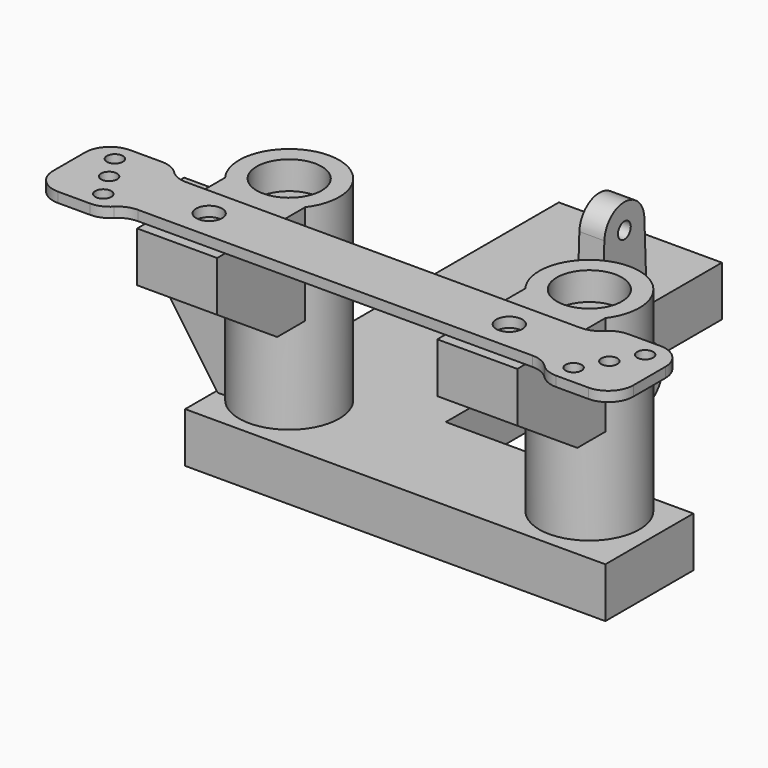
from build123d import *

# Parameters (mm, degrees)
F0_W         = 84
F0_H         = 22
F0_R         = 3
F1_DEPTH     = 10
F3_DEPTH     = 3.2
F6_R         = 4.15
F7_DEPTH     = 20
F8_T1_DEPTH  = 93.5140157162
F9_R         = 7.1
F10_DEPTH    = 12
F12_R        = 1.6
F12_R_2      = 2.6
F13_DEPTH    = 2
F14_T1_DEPTH = 27
F14_T3_DEPTH = 24.9128784748
F15_R        = 5
F17_DEPTH    = 5
F18_R        = 1.6
F19_DEPTH    = 5
F20_R        = 6
F20_R_2      = 1.6
F21_DEPTH    = 3
F22_R        = 4
F23_DEPTH    = 4
F25_DEPTH    = 20
F26_D        = 3.2
F28_W        = 32.6
F28_H        = 69
F29_DEPTH    = 10


# Not quite as in the source:
# - a fillet or chamfer that OpenCascade refuses, or shapes differently, is made with other operations: its cross-section is extruded or revolved along the edge and cut away or added


with BuildPart() as f1:
    # F0 (on Top) → F1 (new body)
    with BuildSketch(Plane.XY):
        Rectangle(F0_W, F0_H)
        with Locations((-30, 0)):
            Circle(F0_R, mode=Mode.SUBTRACT)
        with Locations((30, 0)):
            Circle(F0_R, mode=Mode.SUBTRACT)
    extrude(amount=F1_DEPTH)

    # F2 (on face) → F3 (cut)
    with BuildSketch(Plane.XY.offset(10)):
        Polygon((-25, -2.8867513459), (-25, 2.8867513459), (-30, 5.7735026919), (-35, 2.8867513459), (-35, -2.8867513459), (-30, -5.7735026919), align=None)
        Polygon((25, 2.8867513459), (25, -2.8867513459), (30, -5.7735026919), (35, -2.8867513459), (35, 2.8867513459), (30, 5.7735026919), align=None)
    extrude(amount=-F3_DEPTH, mode=Mode.SUBTRACT)

    # F28 (on face) → F29 (join)
    with BuildSketch(Plane.XY):
        with Locations((-23.8, 45.5)):
            Rectangle(F28_W, F28_H)
    extrude(amount=F29_DEPTH)


with BuildPart() as f5:
    # F4 (on Front) → F5 (revolve)
    with BuildSketch(Plane.XZ):
        Polygon((-40, 50), (-40, 11), (-36.5, 11), (-36.5, 16.6), (-33, 16.6), (-33, 44.4), (-36.5, 44.4), (-36.5, 50), align=None)
    revolve(axis=Axis((-30, 0, 5.9249366093), (0, 0, -1)))

    # F6 (on face) → F7 (join)
    with BuildSketch(Plane.XY.offset(50)):
        with BuildLine():
            ThreePointArc((-22, -6), (-30, -10), (-38, -6))
            Line((-38, -6), (-38, -28))
            Line((-38, -28), (-22, -28))
            Line((-22, -28), (-22, -6))
        make_face()
        with Locations((-30, -20)):
            Circle(F6_R, mode=Mode.SUBTRACT)
    extrude(amount=-F7_DEPTH)

    # F8: chamfer of 10 x 15 on 1 edges, made by hand

    # F8_s2 → F8_t1 (cut)
    with BuildSketch(Plane.YZ.offset(-76.7570078581)):
        Polygon((-13, 30), (-28, 40), (-28, 30), align=None)
    extrude(amount=F8_T1_DEPTH, mode=Mode.SUBTRACT)

    # F9 (on face) → F10 (cut)
    with BuildSketch(Plane(origin=(0, 0, 30), x_dir=(1, 0, 0), z_dir=(0, 0, -1))):
        with Locations((-30, 20)):
            Circle(F9_R)
    extrude(amount=-F10_DEPTH, mode=Mode.SUBTRACT)


with BuildPart() as f11_1:
    # F11: copy of F5
    add(f5.part.moved(Location((60, 0, 0))))


with BuildPart() as f13:
    # F12 (on face) → F13 (new body)
    with BuildSketch(Plane.XY.offset(50)):
        Polygon((0, -26), (42, -26), (42, -29), (58, -29), (58, -11), (42, -11), (42, -14), (0, -14), (-42, -14), (-42, -11), (-58, -11), (-58, -29), (-42, -29), (-42, -26), align=None)
        with Locations((-47, -25.1961524227)):
            Circle(F12_R, mode=Mode.SUBTRACT)
        with Locations((47, -25.1961524227)):
            Circle(F12_R, mode=Mode.SUBTRACT)
        with Locations((-50, -20)):
            Circle(F12_R, mode=Mode.SUBTRACT)
        with Locations((-30, -20)):
            Circle(F12_R_2, mode=Mode.SUBTRACT)
        with Locations((-53, -14.8038475773)):
            Circle(F12_R, mode=Mode.SUBTRACT)
        with Locations((30, -20)):
            Circle(F12_R_2, mode=Mode.SUBTRACT)
        with Locations((50, -20)):
            Circle(F12_R, mode=Mode.SUBTRACT)
        with Locations((53, -14.8038475773)):
            Circle(F12_R, mode=Mode.SUBTRACT)
    extrude(amount=F13_DEPTH)

    # F14: fillet of radius 5 on 8 edges, made by hand

    # F14_s2 → F14_t1 (cut)
    with BuildSketch(Plane.XY.offset(37.5)):
        with BuildLine():
            ThreePointArc((-53, -29), (-56.5355339059, -27.5355339059), (-58, -24))
            Line((-58, -24), (-58, -29))
            Line((-58, -29), (-53, -29))
        make_face()
        with BuildLine():
            ThreePointArc((-58, -16), (-56.5355339059, -12.4644660941), (-53, -11))
            Line((-53, -11), (-58, -11))
            Line((-58, -11), (-58, -16))
        make_face()
        with BuildLine():
            ThreePointArc((58, -24), (56.5355339059, -27.5355339059), (53, -29))
            Line((53, -29), (58, -29))
            Line((58, -29), (58, -24))
        make_face()
        with BuildLine():
            ThreePointArc((53, -11), (56.5355339059, -12.4644660941), (58, -16))
            Line((58, -16), (58, -11))
            Line((58, -11), (53, -11))
        make_face()
    extrude(amount=F14_T1_DEPTH, mode=Mode.SUBTRACT)

    # F14_s4 → F14_t3 (cut)
    with BuildSketch(Plane.XY.offset(38.5435607626)):
        with BuildLine():
            ThreePointArc((-46.582575695, -29), (-43.8439629074, -28.1833001327), (-42, -26))
            Line((-42, -26), (-42, -29))
            Line((-42, -29), (-46.582575695, -29))
        make_face()
        with BuildLine():
            ThreePointArc((-46.582575695, -11), (-43.8439629074, -11.8166998673), (-42, -14))
            Line((-42, -14), (-42, -11))
            Line((-42, -11), (-46.582575695, -11))
        make_face()
        with BuildLine():
            ThreePointArc((46.582575695, -29), (43.8439629074, -28.1833001327), (42, -26))
            Line((42, -26), (42, -29))
            Line((42, -29), (46.582575695, -29))
        make_face()
        with BuildLine():
            ThreePointArc((42, -14), (43.8439629074, -11.8166998673), (46.582575695, -11))
            Line((46.582575695, -11), (42, -11))
            Line((42, -11), (42, -14))
        make_face()
    extrude(amount=F14_T3_DEPTH, mode=Mode.SUBTRACT)

    # F15
    f15_edges = [f13.edges().sort_by_distance(p)[0] for p in [
        (42, -26, 51),
        (42, -14, 51),
        (-42, -14, 51),
        (-42, -26, 51),
    ]]
    fillet(f15_edges, radius=F15_R)


with BuildPart() as f5_1:
    add(f5.part)

    # F16 (on Front) → F17 (join, symmetric)
    with BuildSketch(Plane.XZ):
        Polygon((-40, 32.8592599663), (-45, 40), (-55, 40), (-55, 32), (-40.2956416976, 11), (-37, 11), (-37, 32.8592599663), align=None)
    extrude(amount=F17_DEPTH, both=True)

    # F24 (on face) → F25 (cut)
    with BuildSketch(Plane(origin=(0, 0, 11), x_dir=(1, 0, 0), z_dir=(0, 0, -1))):
        Polygon((-48.4122867597, -2.75), (-46.8245735195, 0), (-48.4122867597, 2.75), (-51.5877132403, 2.75), (-53.1754264805, 0), (-51.5877132403, -2.75), align=None)
    extrude(amount=-F25_DEPTH, mode=Mode.SUBTRACT)

    # F26 (through all)
    with Locations(Plane(origin=(0, 0, 11), x_dir=(1, 0, 0), z_dir=(0, 0, -1))):
        with Locations((-50, 0)):
            Hole(F26_D / 2)


with BuildPart() as f19:
    # F18 (on Right) → F19 (new body)
    with BuildSketch(Plane.YZ):
        with BuildLine():
            Line((45.9951980785, 11.24), (44.9959983987, 36.2))
            ThreePointArc((44.9959983987, 36.2), (40, 41), (35.0040016013, 36.2))
            Line((35.0040016013, 36.2), (34.0048019215, 11.24))
            ThreePointArc((34.0048019215, 11.24), (40, 5), (45.9951980785, 11.24))
        make_face()
        with Locations((40, 11)):
            Circle(F18_R, mode=Mode.SUBTRACT)
        with Locations((40, 36)):
            Circle(F18_R, mode=Mode.SUBTRACT)
    extrude(amount=F19_DEPTH)

    # F20 (on face) → F21 (join)
    with BuildSketch(Plane.YZ.offset(5)):
        with Locations((40, 11)):
            Circle(F20_R)
        with Locations((40, 11)):
            Circle(F20_R_2, mode=Mode.SUBTRACT)
    extrude(amount=F21_DEPTH)

    # F22 (on face) → F23 (cut)
    with BuildSketch(Plane.YZ.offset(8)):
        with Locations((40, 11)):
            Circle(F22_R)
    extrude(amount=-F23_DEPTH, mode=Mode.SUBTRACT)


solid = Compound([f1.part, f11_1.part, f13.part, f5_1.part, f19.part])
